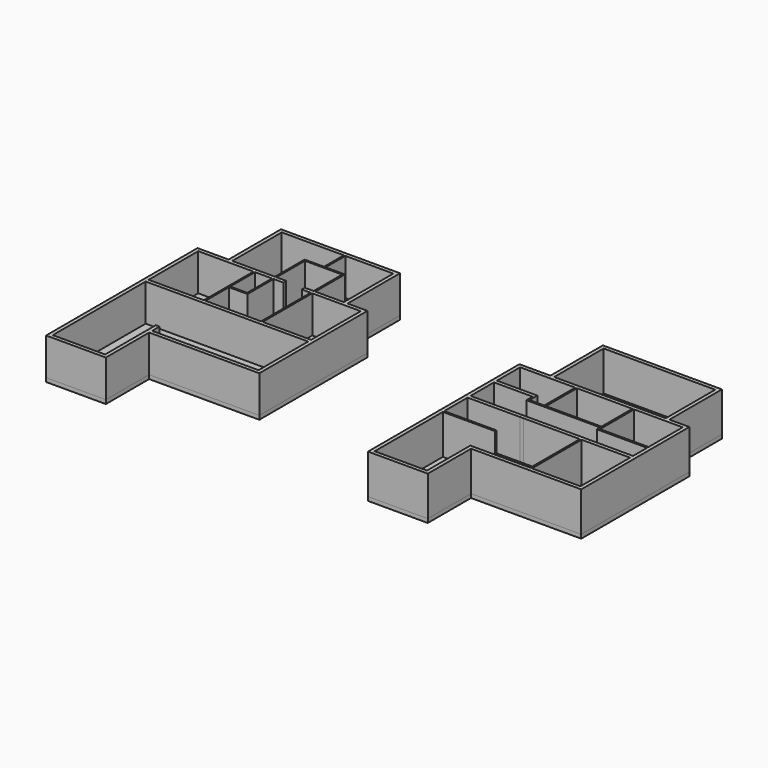
from build123d import *

# Parameters (mm, degrees)
F0_W     = 3.385
F0_H     = 0.24
F0_H_2   = 3.26
F0_W_2   = 0.24
F0_W_3   = 0.1
F0_H_3   = 1.6
F0_H_4   = 0.6
F0_W_4   = 3.575
F0_H_5   = 4.01
F0_W_5   = 3.135
F0_W_6   = 1.2
F0_W_7   = 1.1
F0_H_6   = 2.01
F1_DEPTH = 0.25
F0_H_7   = 0.115
F0_W_8   = 3.635
F0_H_8   = 1.885
F0_W_9   = 0.115
F0_H_9   = 2.76
F2_DEPTH = 2.56
F3_DEPTH = 2.4


with BuildPart() as f1:
    # F0 (on Top) → F1 (new body)
    with BuildSketch(Plane.XY):
        Polygon((-3.4859280568, 4.37), (-5.495, 4.37), (-5.495, -4.37), (-5.255, -4.37), (-5.255, -4.13), (-5.255, -0.12), (-5.255, 0.12), (-5.255, 4.13), (-1.68, 4.13), (-1.58, 4.13), (-0.48, 4.13), (-0.38, 4.13), (0.245, 4.13), (0.245, 4.37), (-0.38, 4.37), (-0.386341276, 4.37), (-0.48, 4.37), (-0.486341276, 4.37), (-3.2459280568, 4.37), align=None)
        Polygon((-3.4859280568, 8.61), (-3.4859280568, 4.37), (-3.2459280568, 4.37), (-3.2459280568, 8.37), (0.77, 8.37), (0.87, 8.37), (3.97, 8.37), (3.97, 4.37), (4.21, 4.37), (4.21, 8.61), align=None)
        Polygon((-5.255, -4.37), (-5.495, -4.37), (-5.495, -7.87), (-1.63, -7.87), (-1.63, -4.37), (-1.87, -4.37), (-1.87, -7.63), (-5.255, -7.63), align=None)
        Polygon((-3.2459280568, 8.37), (-3.2459280568, 4.37), (-0.486341276, 4.37), (-0.486341276, 6.77), (-0.48, 6.77), (0.77, 6.77), (0.77, 8.37), align=None)
        with Locations((-3.5625, -4.25)):
            Rectangle(F0_W, F0_H)
        with Locations((-3.5625, -6)):
            Rectangle(F0_W, F0_H_2)
        Polygon((-0.486341276, 6.77), (-0.486341276, 4.37), (-0.48, 4.37), (-0.386341276, 4.37), (-0.386341276, 6.67), (-0.38, 6.67), (2.02, 6.67), (2.02, 4.37), (2.12, 4.37), (2.12, 6.5391240641), (2.12, 6.77), (0.87, 6.77), (0.77, 6.77), (-0.48, 6.77), align=None)
        with Locations((-1.75, -4.25)):
            Rectangle(F0_W_2, F0_H)
        Polygon((-5.255, -0.12), (-5.255, -4.13), (-1.87, -4.13), (-1.87, -3.53), (-1.63, -3.53), (-1.63, -4.13), (5.255, -4.13), (5.255, -0.12), align=None)
        with Locations((0.82, 7.57)):
            Rectangle(F0_W_3, F0_H_3)
        Polygon((5.495, 4.37), (4.21, 4.37), (3.97, 4.37), (2.12, 4.37), (2.02, 4.37), (1.445, 4.37), (1.445, 4.13), (2.02, 4.13), (2.12, 4.13), (5.255, 4.13), (5.255, 0.12), (5.255, -0.12), (5.255, -4.13), (-1.63, -4.13), (-1.63, -4.37), (5.495, -4.37), align=None)
        with Locations((-1.75, -3.83)):
            Rectangle(F0_W_2, F0_H_4)
        Polygon((-5.255, 0.12), (-5.255, -0.12), (5.255, -0.12), (5.255, 0.12), (2.12, 0.12), (2.02, 0.12), (-1.58, 0.12), (-1.68, 0.12), align=None)
        Polygon((-0.386341276, 6.67), (-0.386341276, 4.37), (-0.38, 4.37), (0.245, 4.37), (1.445, 4.37), (2.02, 4.37), (2.02, 6.67), (-0.38, 6.67), align=None)
        Polygon((3.97, 8.37), (0.87, 8.37), (0.87, 6.77), (2.12, 6.77), (2.12, 6.5391240641), (2.12, 4.37), (3.97, 4.37), align=None)
        with Locations((-3.4675, 2.125)):
            Rectangle(F0_W_4, F0_H_5)
        Polygon((-1.68, 4.13), (-1.68, 0.12), (-1.58, 0.12), (-1.58, 2.02), (-1.58, 2.12), (-1.58, 4.13), align=None)
        with Locations((3.6875, 2.125)):
            Rectangle(F0_W_5, F0_H_5)
        with Locations((0.845, 4.25)):
            Rectangle(F0_W_6, F0_H)
        Polygon((-1.58, 2.02), (-1.58, 0.12), (2.02, 0.12), (2.02, 4.13), (1.445, 4.13), (0.245, 4.13), (-0.38, 4.13), (-0.38, 2.02), align=None)
        with Locations((2.07, 2.125)):
            Rectangle(F0_W_3, F0_H_5)
        with Locations((-1.03, 3.125)):
            Rectangle(F0_W_7, F0_H_6)
        Polygon((-1.58, 2.12), (-1.58, 2.02), (-0.38, 2.02), (-0.38, 4.13), (-0.48, 4.13), (-0.48, 2.12), align=None)
    extrude(amount=-F1_DEPTH)


with BuildPart() as f1b:
    # F0 (on Top) → F1, piece 2 (new body)
    with BuildSketch(Plane.XY):
        Polygon((17.3313135152, 4.37), (15.3252581853, 4.37), (15.3252581853, -4.37), (15.5652581853, -4.37), (15.5652581853, -4.13), (15.5652581853, -2.12), (15.5652581853, -2.005), (15.5652581853, -0.12), (15.5652581853, 0.12), (15.5652581853, 2.015), (15.5652581853, 2.255), (15.5652581853, 4.13), (19.1252581853, 4.13), (19.1402581853, 4.13), (19.2402581853, 4.13), (20.3402581853, 4.13), (20.4402581853, 4.13), (22.8252581853, 4.13), (22.8402581853, 4.13), (22.9402581853, 4.13), (26.0752581853, 4.13), (26.0752581853, 1.37), (26.0752581853, 1.255), (26.0752581853, 0.12), (26.0752581853, -0.12), (26.0752581853, -4.13), (22.9402581853, -4.13), (22.8252581853, -4.13), (19.1902581853, -4.13), (19.1902581853, -4.37), (26.3152581853, -4.37), (26.3152581853, 4.37), (25.0302581853, 4.37), (24.7902581853, 4.37), (20.437241572, 4.37), (20.430900296, 4.37), (20.3402581853, 4.37), (20.330900296, 4.37), (17.5713135152, 4.37), align=None)
        Polygon((17.3313135152, 8.61), (17.3313135152, 4.37), (17.5713135152, 4.37), (17.5713135152, 8.37), (21.587241572, 8.37), (21.6902581853, 8.37), (24.7902581853, 8.37), (24.7902581853, 4.37), (25.0302581853, 4.37), (25.0302581853, 8.61), align=None)
        Polygon((15.5652581853, -4.37), (15.3252581853, -4.37), (15.3252581853, -7.87), (19.1902581853, -7.87), (19.1902581853, -4.37), (18.9502581853, -4.37), (18.9502581853, -7.63), (15.5652581853, -7.63), align=None)
        Polygon((17.5713135152, 8.37), (17.5713135152, 4.37), (20.330900296, 4.37), (20.3402581853, 4.37), (20.430900296, 4.37), (20.437241572, 4.37), (24.7902581853, 4.37), (24.7902581853, 8.37), (21.6902581853, 8.37), (21.587241572, 8.37), align=None)
        with Locations((17.2577581853, -4.25)):
            Rectangle(F0_W, F0_H)
        with Locations((17.2577581853, -6)):
            Rectangle(F0_W, F0_H_2)
        with Locations((19.0702581853, -4.25)):
            Rectangle(F0_W_2, F0_H)
        with Locations((17.2577581853, -3.125)):
            Rectangle(F0_W, F0_H_6)
        Polygon((18.9502581853, -2.12), (18.9502581853, -4.13), (19.1902581853, -4.13), (19.1902581853, -0.12), (18.9502581853, -0.12), (18.9502581853, -2.005), align=None)
        with Locations((17.2577581853, -2.0625)):
            Rectangle(F0_W, F0_H_7)
        with Locations((21.0077581853, -2.125)):
            Rectangle(F0_W_8, F0_H_5)
        with Locations((17.2577581853, -1.0625)):
            Rectangle(F0_W, F0_H_8)
        with Locations((22.8827581853, -2.125)):
            Rectangle(F0_W_9, F0_H_5)
        Polygon((19.1902581853, -0.1174762056), (19.1902581853, -0.12), (22.8252581853, -0.12), (22.9402581853, -0.12), (26.0752581853, -0.12), (26.0752581853, 0.12), (22.9402581853, 0.12), (22.8402581853, 0.12), (19.2402581853, 0.12), (19.1402581853, 0.12), (15.5652581853, 0.12), (15.5652581853, -0.12), (18.9502581853, -0.12), (18.9502581853, -0.1174762056), align=None)
        with Locations((24.5077581853, -2.125)):
            Rectangle(F0_W_5, F0_H_5)
        Polygon((15.5652581853, 2.015), (15.5652581853, 0.12), (19.1402581853, 0.12), (19.2402581853, 0.12), (22.8402581853, 0.12), (22.9402581853, 0.12), (26.0752581853, 0.12), (26.0752581853, 1.255), (22.8252581853, 1.255), (22.8252581853, 1.5153254153), (18.0602581853, 1.5153254153), (18.0602581853, 2.015), align=None)
        Polygon((15.5652581853, 2.255), (15.5652581853, 2.015), (18.0602581853, 2.015), (18.0602581853, 1.5153254153), (22.8252581853, 1.5153254153), (22.8252581853, 1.6303254153), (19.2402581853, 1.6303254153), (19.1252581853, 1.6303254153), (18.1752581853, 1.6303254153), (18.1752581853, 2.255), align=None)
        Polygon((15.5652581853, 4.13), (15.5652581853, 2.255), (18.1752581853, 2.255), (18.1752581853, 1.6303254153), (19.1252581853, 1.6303254153), (19.1252581853, 4.13), align=None)
        Polygon((22.8252581853, 1.255), (26.0752581853, 1.255), (26.0752581853, 1.37), (22.9402581853, 1.37), (22.9402581853, 4.13), (22.8402581853, 4.13), (22.8252581853, 4.13), (22.8252581853, 1.6303254153), (22.8252581853, 1.5153254153), align=None)
        Polygon((19.1402581853, 4.13), (19.1252581853, 4.13), (19.1252581853, 1.6303254153), (19.2402581853, 1.6303254153), (19.2402581853, 4.13), align=None)
        with Locations((24.5077581853, 2.75)):
            Rectangle(F0_W_5, F0_H_9)
        Polygon((19.2402581853, 1.6303254153), (22.8252581853, 1.6303254153), (22.8252581853, 4.13), (20.4402581853, 4.13), (20.3402581853, 4.13), (19.2402581853, 4.13), align=None)
    extrude(amount=-F1_DEPTH)


with BuildPart() as f2:
    # F0 (on Top) → F2 (new body)
    with BuildSketch(Plane.XY):
        Polygon((17.3313135152, 4.37), (15.3252581853, 4.37), (15.3252581853, -4.37), (15.5652581853, -4.37), (15.5652581853, -4.13), (15.5652581853, -2.12), (15.5652581853, -2.005), (15.5652581853, -0.12), (15.5652581853, 0.12), (15.5652581853, 2.015), (15.5652581853, 2.255), (15.5652581853, 4.13), (19.1252581853, 4.13), (19.1402581853, 4.13), (19.2402581853, 4.13), (20.3402581853, 4.13), (20.4402581853, 4.13), (22.8252581853, 4.13), (22.8402581853, 4.13), (22.9402581853, 4.13), (26.0752581853, 4.13), (26.0752581853, 1.37), (26.0752581853, 1.255), (26.0752581853, 0.12), (26.0752581853, -0.12), (26.0752581853, -4.13), (22.9402581853, -4.13), (22.8252581853, -4.13), (19.1902581853, -4.13), (19.1902581853, -4.37), (26.3152581853, -4.37), (26.3152581853, 4.37), (25.0302581853, 4.37), (24.7902581853, 4.37), (20.437241572, 4.37), (20.430900296, 4.37), (20.3402581853, 4.37), (20.330900296, 4.37), (17.5713135152, 4.37), align=None)
        Polygon((15.5652581853, 2.255), (15.5652581853, 2.015), (18.0602581853, 2.015), (18.0602581853, 1.5153254153), (22.8252581853, 1.5153254153), (22.8252581853, 1.6303254153), (19.2402581853, 1.6303254153), (19.1252581853, 1.6303254153), (18.1752581853, 1.6303254153), (18.1752581853, 2.255), align=None)
        with Locations((19.0702581853, -4.25)):
            Rectangle(F0_W_2, F0_H)
        Polygon((19.1402581853, 4.13), (19.1252581853, 4.13), (19.1252581853, 1.6303254153), (19.2402581853, 1.6303254153), (19.2402581853, 4.13), align=None)
        Polygon((22.8252581853, 1.255), (26.0752581853, 1.255), (26.0752581853, 1.37), (22.9402581853, 1.37), (22.9402581853, 4.13), (22.8402581853, 4.13), (22.8252581853, 4.13), (22.8252581853, 1.6303254153), (22.8252581853, 1.5153254153), align=None)
        with Locations((22.8827581853, -2.125)):
            Rectangle(F0_W_9, F0_H_5)
        Polygon((19.1902581853, -0.1174762056), (19.1902581853, -0.12), (22.8252581853, -0.12), (22.9402581853, -0.12), (26.0752581853, -0.12), (26.0752581853, 0.12), (22.9402581853, 0.12), (22.8402581853, 0.12), (19.2402581853, 0.12), (19.1402581853, 0.12), (15.5652581853, 0.12), (15.5652581853, -0.12), (18.9502581853, -0.12), (18.9502581853, -0.1174762056), align=None)
        with Locations((17.2577581853, -2.0625)):
            Rectangle(F0_W, F0_H_7)
        Polygon((15.5652581853, -4.37), (15.3252581853, -4.37), (15.3252581853, -7.87), (19.1902581853, -7.87), (19.1902581853, -4.37), (18.9502581853, -4.37), (18.9502581853, -7.63), (15.5652581853, -7.63), align=None)
        Polygon((17.3313135152, 8.61), (17.3313135152, 4.37), (17.5713135152, 4.37), (17.5713135152, 8.37), (21.587241572, 8.37), (21.6902581853, 8.37), (24.7902581853, 8.37), (24.7902581853, 4.37), (25.0302581853, 4.37), (25.0302581853, 8.61), align=None)
    extrude(amount=F2_DEPTH)


with BuildPart() as f3:
    # F0 (on Top) → F3 (new body)
    with BuildSketch(Plane.XY):
        Polygon((-3.4859280568, 8.61), (-3.4859280568, 4.37), (-3.2459280568, 4.37), (-3.2459280568, 8.37), (0.77, 8.37), (0.87, 8.37), (3.97, 8.37), (3.97, 4.37), (4.21, 4.37), (4.21, 8.61), align=None)
        Polygon((5.495, 4.37), (4.21, 4.37), (3.97, 4.37), (2.12, 4.37), (2.02, 4.37), (1.445, 4.37), (1.445, 4.13), (2.02, 4.13), (2.12, 4.13), (5.255, 4.13), (5.255, 0.12), (5.255, -0.12), (5.255, -4.13), (-1.63, -4.13), (-1.63, -4.37), (5.495, -4.37), align=None)
        Polygon((-3.4859280568, 4.37), (-5.495, 4.37), (-5.495, -4.37), (-5.255, -4.37), (-5.255, -4.13), (-5.255, -0.12), (-5.255, 0.12), (-5.255, 4.13), (-1.68, 4.13), (-1.58, 4.13), (-0.48, 4.13), (-0.38, 4.13), (0.245, 4.13), (0.245, 4.37), (-0.38, 4.37), (-0.386341276, 4.37), (-0.48, 4.37), (-0.486341276, 4.37), (-3.2459280568, 4.37), align=None)
        Polygon((-5.255, -4.37), (-5.495, -4.37), (-5.495, -7.87), (-1.63, -7.87), (-1.63, -4.37), (-1.87, -4.37), (-1.87, -7.63), (-5.255, -7.63), align=None)
        with Locations((-1.75, -4.25)):
            Rectangle(F0_W_2, F0_H)
        with Locations((-1.75, -3.83)):
            Rectangle(F0_W_2, F0_H_4)
        Polygon((-5.255, 0.12), (-5.255, -0.12), (5.255, -0.12), (5.255, 0.12), (2.12, 0.12), (2.02, 0.12), (-1.58, 0.12), (-1.68, 0.12), align=None)
        Polygon((-1.68, 4.13), (-1.68, 0.12), (-1.58, 0.12), (-1.58, 2.02), (-1.58, 2.12), (-1.58, 4.13), align=None)
        with Locations((2.07, 2.125)):
            Rectangle(F0_W_3, F0_H_5)
        Polygon((-1.58, 2.12), (-1.58, 2.02), (-0.38, 2.02), (-0.38, 4.13), (-0.48, 4.13), (-0.48, 2.12), align=None)
        Polygon((-0.486341276, 6.77), (-0.486341276, 4.37), (-0.48, 4.37), (-0.386341276, 4.37), (-0.386341276, 6.67), (-0.38, 6.67), (2.02, 6.67), (2.02, 4.37), (2.12, 4.37), (2.12, 6.5391240641), (2.12, 6.77), (0.87, 6.77), (0.77, 6.77), (-0.48, 6.77), align=None)
        with Locations((0.82, 7.57)):
            Rectangle(F0_W_3, F0_H_3)
    extrude(amount=F3_DEPTH)


solid = Compound([f1.part, f1b.part, f2.part, f3.part])
